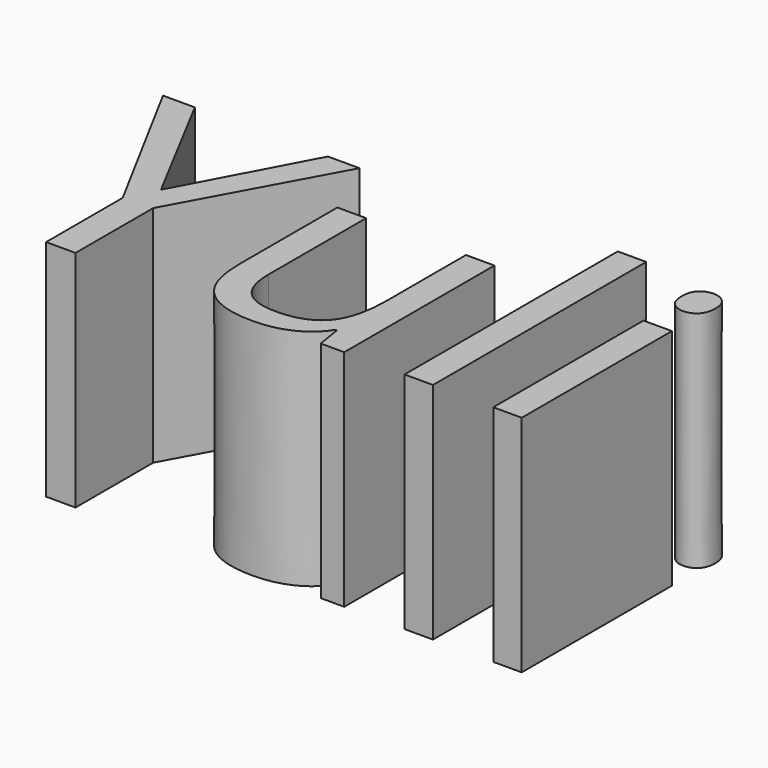
from build123d import *

# Parameters (mm, degrees)
F0_TEXT_SIZE = 39.7454358689
F1_DEPTH     = 25.4


# Not quite as in the source:
# - Text() gives the source's letters only with a copy of the font that has no kerning and outlines rounded to 1/6400 em; it was checked with that copy


with BuildPart() as f1:
    # F0 (on Top) → F1 (new body)
    with BuildSketch(Plane.XY):
        with Locations((-16.4497438818, 6.1321533285)):
            Text('Yuli', F0_TEXT_SIZE, font='Open Sans', text_align=(TextAlign.LEFT, TextAlign.BOTTOM))
    extrude(amount=F1_DEPTH)


solid = f1.part
